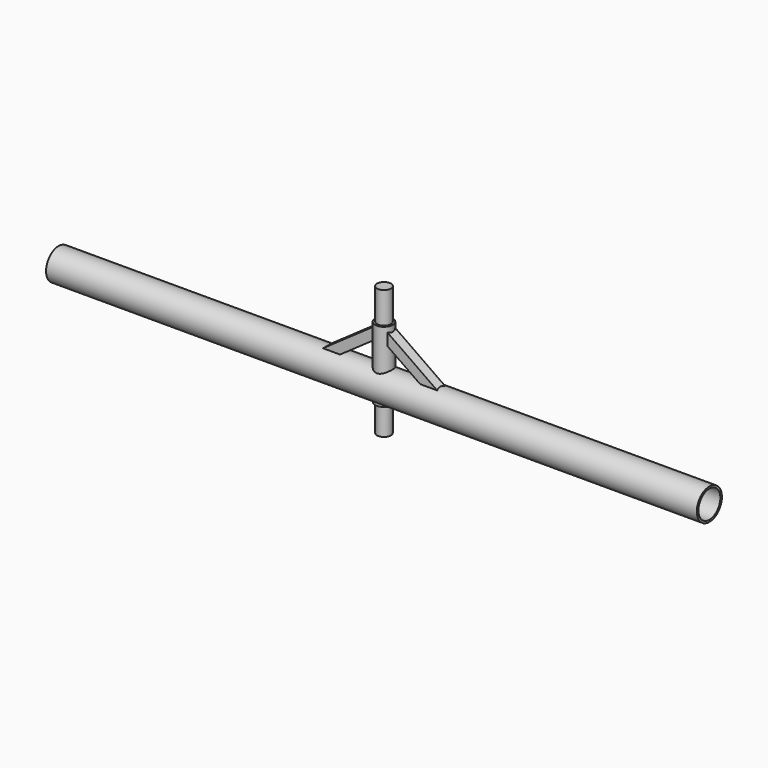
from build123d import *

# Parameters (mm, degrees)
F0_R          = 40
F1_DEPTH      = 830
F1_DEPTH_BACK = 830
F2_R          = 22.5
F3_DEPTH      = 140
F3_DEPTH_BACK = 40
F4_R          = 17.5
F5_DEPTH      = 80
F5_DEPTH_BACK = 250
F7_DEPTH      = 12.5
F8_R          = 35.000000149
F9_DEPTH      = 1660.0010001


# Not quite as in the source:
# - a pattern or mirror of a feature is missing from the dataset's text; its kind, count and spacing are read off the source's solid


with BuildPart() as f1:
    # F0 (on Right) → F1 (new body, two sides)
    with BuildSketch(Plane.YZ) as f1_sk:
        Circle(F0_R)
    extrude(amount=F1_DEPTH)
    extrude(f1_sk.sketch, amount=-F1_DEPTH_BACK)

    # F2 (on Top) → F3 (join, two sides)
    with BuildSketch(Plane.XY) as f3_sk:
        Circle(F2_R)
    extrude(amount=F3_DEPTH)
    extrude(f3_sk.sketch, amount=-F3_DEPTH_BACK)

    # F4 (on face) → F5 (join, two sides)
    with BuildSketch(Plane.XY.offset(140)) as f5_sk:
        Circle(F4_R)
    extrude(amount=F5_DEPTH)
    extrude(f5_sk.sketch, amount=-F5_DEPTH_BACK)

    # F6 (on Front) → F7 (join, symmetric)
    with BuildSketch(Plane.XZ):
        Polygon((0, 109.4836109607), (0, 140), (-200, 0), (-156.4051585152, 0), align=None)
    f7 = extrude(amount=F7_DEPTH, both=True)

    # F7_copies: F7 across plane
    add(f7.mirror(Plane(origin=(0, 0, 0), x_dir=(0, 0, 1), z_dir=(1, 0, 0))))

    # F8 (on face) → F9 (cut, through all)
    with BuildSketch(Plane(origin=(-830, 0, 0), x_dir=(0, -1, 0), z_dir=(-1, 0, 0))):
        Circle(F8_R)
    extrude(amount=-F9_DEPTH, mode=Mode.SUBTRACT)


solid = f1.part
